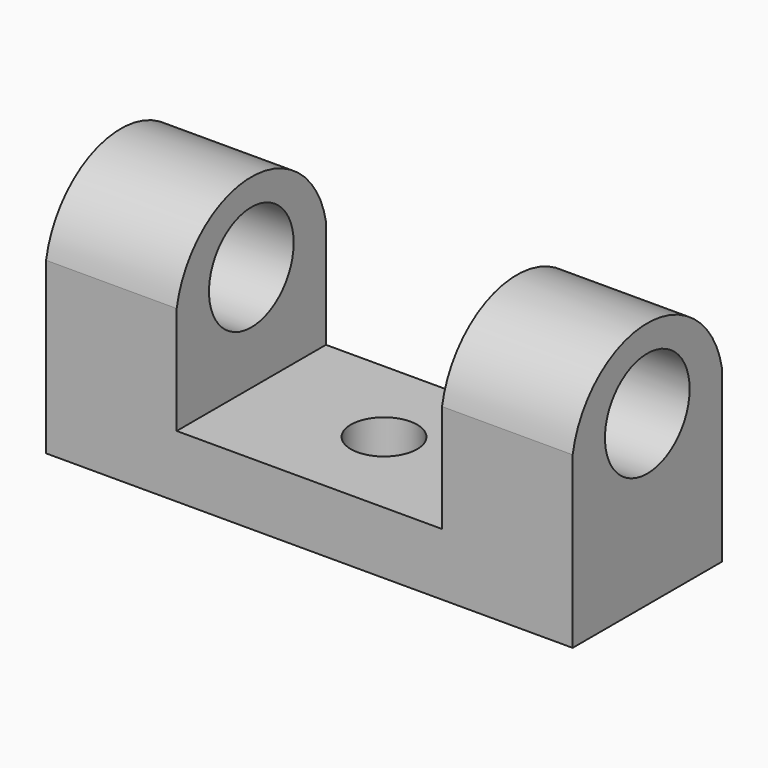
from build123d import *

# Parameters (mm, degrees)
F0_W     = 25.4
F0_H     = 9
F1_DEPTH = 3
F2_W     = 6.3
F2_H     = 9
F3_DEPTH = 9
F5_DEPTH = 25
F6_DEPTH = 25
F8_D     = 5.1054
F9_D     = 3.2


with BuildPart() as f1:
    # F0 (on Top) → F1 (new body)
    with BuildSketch(Plane.XY):
        Rectangle(F0_W, F0_H)
    extrude(amount=F1_DEPTH)

    # F2 (on face) → F3 (join)
    with BuildSketch(Plane.XY.offset(3)):
        with Locations((-9.55, 0)):
            Rectangle(F2_W, F2_H)
        with Locations((9.55, 0)):
            Rectangle(F2_W, F2_H)
    extrude(amount=F3_DEPTH)

    # F4 (on face) → F5 (cut)
    with BuildSketch(Plane.YZ.offset(12.7)):
        with BuildLine():
            ThreePointArc((-4.5, 8.2006715238), (-0.0114142109, 11.9599530691), (4.5, 8.2280980423))
            Line((4.5, 8.2280980423), (4.5, 12))
            Line((4.5, 12), (-4.5, 12))
            Line((-4.5, 12), (-4.5, 8.2006715238))
        make_face()
    extrude(amount=-F5_DEPTH, mode=Mode.SUBTRACT)

    # F6 (cut): a face of the model
    f6_faces = [f1.faces().sort_by_distance(p)[0] for p in [
        (-12.3, -0.0114439809, 11.9697221024),
    ]]
    extrude(f6_faces, amount=-F6_DEPTH, mode=Mode.SUBTRACT)

    # F8 (through all)
    with Locations(Plane(origin=(-12.7, 0, 0), x_dir=(0, -1, 0), z_dir=(-1, 0, 0))):
        with Locations((0, 8.1223854795)):
            Hole(F8_D / 2)

    # F9 (through all)
    with Locations(Plane(origin=(0, 0, 0), x_dir=(1, 0, 0), z_dir=(0, 0, -1))):
        with Locations((0, 0)):
            Hole(F9_D / 2)


solid = f1.part
